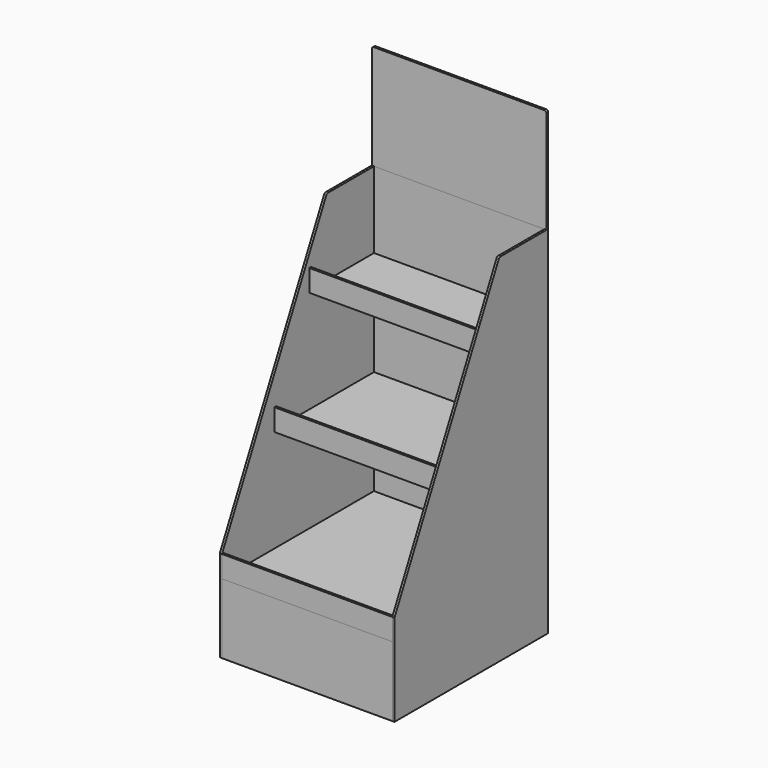
from build123d import *

# Parameters (mm, degrees)
F1_DEPTH  = 6.35
F2_W      = 508
F2_H      = 1034.8848681509
F3_DEPTH  = 6.35
F7_W      = 495.3
F7_H      = 203.2776648521
F8_DEPTH  = 6.35
F9_W      = 495.3
F9_H      = 546.1
F10_DEPTH = 6.35
F12_W     = 495.3
F12_H     = 355.6
F13_DEPTH = 6.35
F14_W     = 495.3
F14_H     = 63.5
F15_DEPTH = 6.35
F17_W     = 495.3
F17_H     = 228.6
F18_DEPTH = 6.35
F19_W     = 495.3
F19_H     = 63.5
F20_DEPTH = 6.35
F21_W     = 508
F21_H     = 6.35
F22_DEPTH = 304.8
F23_R     = 6.35
F24_W     = 161.925
F24_H     = 6.35
F24_W_2   = 6.35
F24_H_2   = 178.689
F24_W_3   = 158.75
F24_H_3   = 175.514
F24_H_4   = 179.197
F25_DEPTH = 196.9276648521
F26_W     = 495.3
F26_H     = 6.35
F27_DEPTH = 63.4223351
F28_R     = 6.35
F28_2_R   = 6.35


# Not quite as in the source:
# - an extrude ends at something that could not be found from the text; its depth is read off the source's solid


with BuildPart() as f1:
    # F0 (on Right) → F1 (new body)
    with BuildSketch(Plane.YZ):
        Polygon((-313.6506947781, 123.2482513189), (-313.6506947781, -79.9517486811), (245.1493052219, -79.9517486811), (245.1493052219, 954.9331194699), (67.3493052219, 954.9331194699), (-313.6506947781, 186.7482513189), align=None)
    extrude(amount=F1_DEPTH)


with BuildPart() as f3:
    # F2 (on face) → F3 (new body)
    with BuildSketch(Plane(origin=(0, 245.1493052219, 0), x_dir=(-1, 0, 0), z_dir=(0, 1, 0))):
        with Locations((247.65, 437.4906853944)):
            Rectangle(F2_W, F2_H)
    extrude(amount=-F3_DEPTH)


with BuildPart() as f6_1:
    # F6: instance of F1
    add(f1.part.mirror(Plane.YZ.offset(-247.65)))

    # F28#2
    f28_2_edges = [f6_1.edges().sort_by_distance(p)[0] for p in [
        (-498.475, 67.349305, 954.933119),
    ]]
    fillet(f28_2_edges, radius=F28_2_R)


with BuildPart() as f8:
    # F7 (on face) → F8 (new body)
    with BuildSketch(Plane.XZ.offset(313.6506947781)):
        with Locations((-247.65, 21.687083745)):
            Rectangle(F7_W, F7_H)
    extrude(amount=-F8_DEPTH)


with BuildPart() as f10:
    # F9 (on face) → F10 (new body)
    with BuildSketch(Plane.XY.offset(123.3259161711)):
        with Locations((-247.65, -34.2506947781)):
            Rectangle(F9_W, F9_H)
    extrude(amount=-F10_DEPTH)


with BuildPart() as f13:
    # F12 (on plane+point) → F13 (new body)
    with BuildSketch(Plane.XY.offset(428.0482513189)):
        with Locations((-247.65, 60.9993052219)):
            Rectangle(F12_W, F12_H)
    extrude(amount=-F13_DEPTH)


with BuildPart() as f15:
    # F14 (on face) → F15 (new body)
    with BuildSketch(Plane.XZ.offset(116.8006947781)):
        with Locations((-247.65, 453.4482513189)):
            Rectangle(F14_W, F14_H)
    extrude(amount=F15_DEPTH)


with BuildPart() as f18:
    # F17 (on plane+point) → F18 (new body)
    with BuildSketch(Plane.XY.offset(732.8482513189)):
        with Locations((-247.65, 124.4993052219)):
            Rectangle(F17_W, F17_H)
    extrude(amount=-F18_DEPTH)


with BuildPart() as f20:
    # F19 (on face) → F20 (new body)
    with BuildSketch(Plane.XZ.offset(-10.1993052219)):
        with Locations((-247.65, 758.2482513189)):
            Rectangle(F19_W, F19_H)
    extrude(amount=F20_DEPTH)


with BuildPart() as f22:
    # F21 (on face) → F22 (new body)
    with BuildSketch(Plane.XY.offset(954.9331194699)):
        with Locations((-247.65, 241.9743052219)):
            Rectangle(F21_W, F21_H)
    extrude(amount=F22_DEPTH)

    # F23
    f23_edges = [f22.edges().sort_by_distance(p)[0] for p in [
        (6.35, 241.974305, 1259.733119),
        (-501.65, 241.974305, 1259.733119),
    ]]
    fillet(f23_edges, radius=F23_R)


with BuildPart() as f25:
    # F24 (on face) → F25 (new body, through all)
    with BuildSketch(Plane(origin=(0, 0, 116.9759161711), x_dir=(1, 0, 0), z_dir=(0, 0, -1))):
        with Locations((-80.9625, 125.4366947781)):
            Rectangle(F24_W, F24_H)
        with Locations((-165.1, 125.4366947781)):
            Rectangle(F24_W_2, F24_H)
        with Locations((-165.1, 217.9561947781)):
            Rectangle(F24_W_2, F24_H_2)
        with Locations((-247.65, 125.4366947781)):
            Rectangle(F24_W_3, F24_H)
        with Locations((-165.1, 34.5046947781)):
            Rectangle(F24_W_2, F24_H_3)
        with Locations((-330.2, 125.4366947781)):
            Rectangle(F24_W_2, F24_H)
        with Locations((-330.2, 217.9561947781)):
            Rectangle(F24_W_2, F24_H_2)
        with Locations((-165.1, -56.4273052219)):
            Rectangle(F24_W_2, F24_H)
        with Locations((-80.9625, -56.4273052219)):
            Rectangle(F24_W, F24_H)
        with Locations((-414.3375, 125.4366947781)):
            Rectangle(F24_W, F24_H)
        with Locations((-330.2, 34.5046947781)):
            Rectangle(F24_W_2, F24_H_3)
        with Locations((-247.65, -56.4273052219)):
            Rectangle(F24_W_3, F24_H)
        with Locations((-165.1, -149.2008052219)):
            Rectangle(F24_W_2, F24_H_4)
        with Locations((-330.2, -56.4273052219)):
            Rectangle(F24_W_2, F24_H)
        with Locations((-414.3375, -56.4273052219)):
            Rectangle(F24_W, F24_H)
        with Locations((-330.2, -149.2008052219)):
            Rectangle(F24_W_2, F24_H_4)
    extrude(amount=F25_DEPTH)


with BuildPart() as f27:
    # F26 (on face) → F27 (new body, through all)
    with BuildSketch(Plane.XY.offset(123.3259161711)):
        with Locations((-247.65, -310.4756947781)):
            Rectangle(F26_W, F26_H)
    extrude(amount=F27_DEPTH)


with BuildPart() as f1_1:
    add(f1.part)

    # F28
    f28_edges = [f1_1.edges().sort_by_distance(p)[0] for p in [
        (3.175, 67.349305, 954.933119),
    ]]
    fillet(f28_edges, radius=F28_R)


solid = Compound([f3.part, f6_1.part, f8.part, f10.part, f13.part, f15.part, f18.part, f20.part, f22.part, f25.part, f27.part, f1_1.part])
